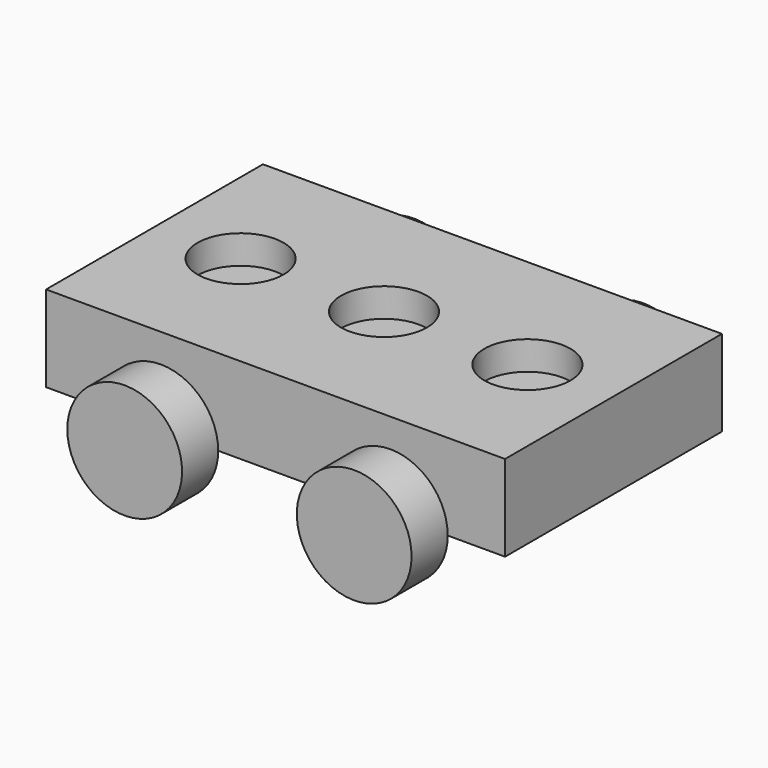
from build123d import *

# Parameters (mm, degrees)
F0_W     = 101.6
F0_H     = 60
F1_DEPTH = 19.05
F2_R     = 9.525
F3_DEPTH = 6.35
F5_DEPTH = 10


# Not quite as in the source:
# - a length typed as a fraction of an inch, garbled in the dataset ("3 / 203.2 mm" for 3/8 in), is restored


with BuildPart() as f1:
    # F0 (on Top) → F1 (new body)
    with BuildSketch(Plane.XY):
        Rectangle(F0_W, F0_H)
    extrude(amount=F1_DEPTH)

    # F2 (on face) → F3 (cut)
    with BuildSketch(Plane.XY.offset(19.05)):
        Circle(F2_R)
        with Locations((31.75, 0)):
            Circle(F2_R)
        with Locations((-31.75, 0)):
            Circle(F2_R)
    extrude(amount=-F3_DEPTH, mode=Mode.SUBTRACT)

    # F4 (on face) → F5 (join)
    with BuildSketch(Plane(origin=(0, 30, 0), x_dir=(-1, 0, 0), z_dir=(0, 1, 0))):
        with BuildLine():
            ThreePointArc((-12.7, 0), (-25.4, 12.7), (-38.1, 0))
            Line((-38.1, 0), (-25.4, 0))
            Line((-25.4, 0), (-12.7, 0))
        make_face()
        with BuildLine():
            Line((-25.4, 0), (-38.1, 0))
            ThreePointArc((-38.1, 0), (-25.4, -12.7), (-12.7, 0))
            Line((-12.7, 0), (-25.4, 0))
        make_face()
    extrude(amount=F5_DEPTH)


with BuildPart() as f6_1:
    # F6: instance of F1
    add(f1.part.mirror(Plane.YZ))


with BuildPart() as f1_1:
    add(f1.part)

    add(f6_1.part)  # F7 merges F6_1
    # F7: F6_1, F1 across plane
    add(f6_1.part.mirror(Plane.XZ))
    add(f1.part.mirror(Plane.XZ))


solid = f1_1.part
